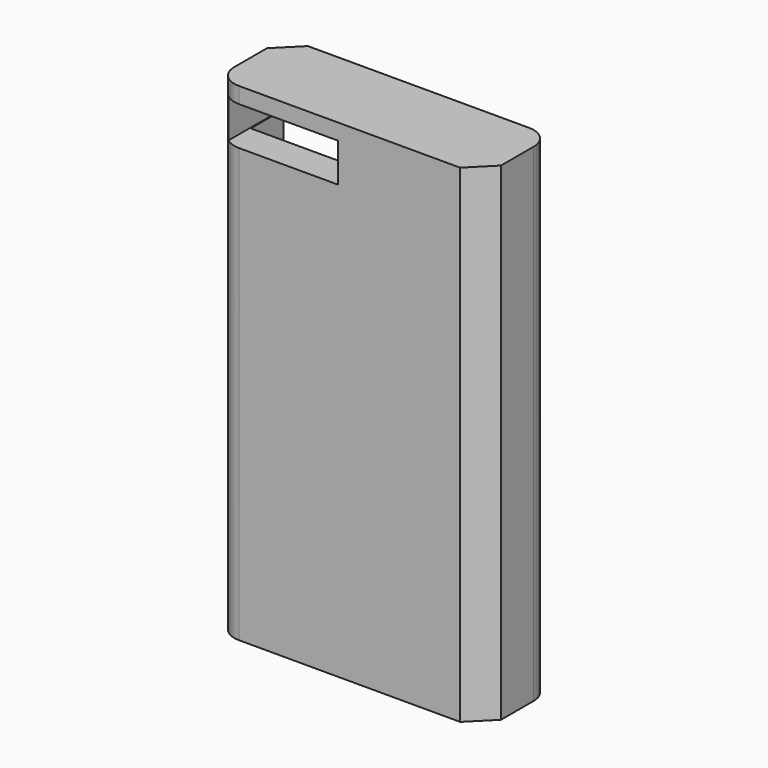
from build123d import *

# Parameters (mm, degrees)
F0_W         = 59.69
F0_H         = 109.22
F1_DEPTH     = 19.304
F2_W         = 50.8
F2_H         = 100.838
F3_DEPTH     = 12.192
F4_W         = 5.1237940788
F4_H         = 100.838
F5_DEPTH     = 12.192
F6_W         = 25.4
F6_H         = 8.6614
F7_DEPTH     = 45.974
F8_T1_DEPTH  = 134.62
F9_SIZE      = 5.08
F10_T1_DEPTH = 134.62
F11_T1_DEPTH = 135.3482991577


# Not quite as in the source:
# - a fillet or chamfer that OpenCascade refuses, or shapes differently, is made with other operations: its cross-section is extruded or revolved along the edge and cut away or added


with BuildPart() as f1:
    # F0 (on Front) → F1 (new body)
    with BuildSketch(Plane.XZ):
        with Locations((1.3794824481, 0)):
            Rectangle(F0_W, F0_H)
    extrude(amount=F1_DEPTH)

    # F2 (on Front) → F3 (cut)
    with BuildSketch(Plane.XZ):
        with Locations((3.9194825381, 1.5458958449)):
            Rectangle(F2_W, F2_H)
    extrude(amount=F3_DEPTH, mode=Mode.SUBTRACT)

    # F4 (on Front) → F5 (cut)
    with BuildSketch(Plane.XZ):
        with Locations((-23.8453447819, 1.9400352838)):
            Rectangle(F4_W, F4_H)
    extrude(amount=F5_DEPTH, mode=Mode.SUBTRACT)

    # F6 (on Front) → F7 (cut)
    with BuildSketch(Plane.XZ):
        with Locations((-13.9043106094, 46.7005276281)):
            Rectangle(F6_W, F6_H)
    extrude(amount=F7_DEPTH, mode=Mode.SUBTRACT)

    # F8: fillet of radius 5.08 on 1 edges, made by hand

    # F8_s2 → F8_t1 (cut)
    with BuildSketch(Plane.XY.offset(-67.31)):
        with BuildLine():
            ThreePointArc((-28.4655175519, -14.224), (-26.9776200003, -17.8161024484), (-23.3855175519, -19.304))
            Line((-23.3855175519, -19.304), (-28.4655175519, -19.304))
            Line((-28.4655175519, -19.304), (-28.4655175519, -14.224))
        make_face()
    extrude(amount=F8_T1_DEPTH, mode=Mode.SUBTRACT)

    # F9
    f9_edges = [f1.edges().sort_by_distance(p)[0] for p in [
        (31.224482, -19.304, 0),
    ]]
    chamfer(f9_edges, length=F9_SIZE)

    # F10: fillet of radius 5.08 on 1 edges, made by hand

    # F10_s2 → F10_t1 (cut)
    with BuildSketch(Plane.XY.offset(-67.31)):
        with BuildLine():
            ThreePointArc((31.2244824481, -5.08), (29.7365848965, -1.4878975516), (26.1444824481, 0))
            Line((26.1444824481, 0), (31.2244824481, 0))
            Line((31.2244824481, 0), (31.2244824481, -5.08))
        make_face()
    extrude(amount=F10_T1_DEPTH, mode=Mode.SUBTRACT)

    # F11: chamfer of 5.08 on 1 edges, made by hand

    # F11_s2 → F11_t1 (cut)
    with BuildSketch(Plane.XY.offset(-67.6741495789)):
        Polygon((-28.4655175519, -5.08), (-23.3855175519, 0), (-28.4655175519, 0), align=None)
    extrude(amount=F11_T1_DEPTH, mode=Mode.SUBTRACT)


solid = f1.part
